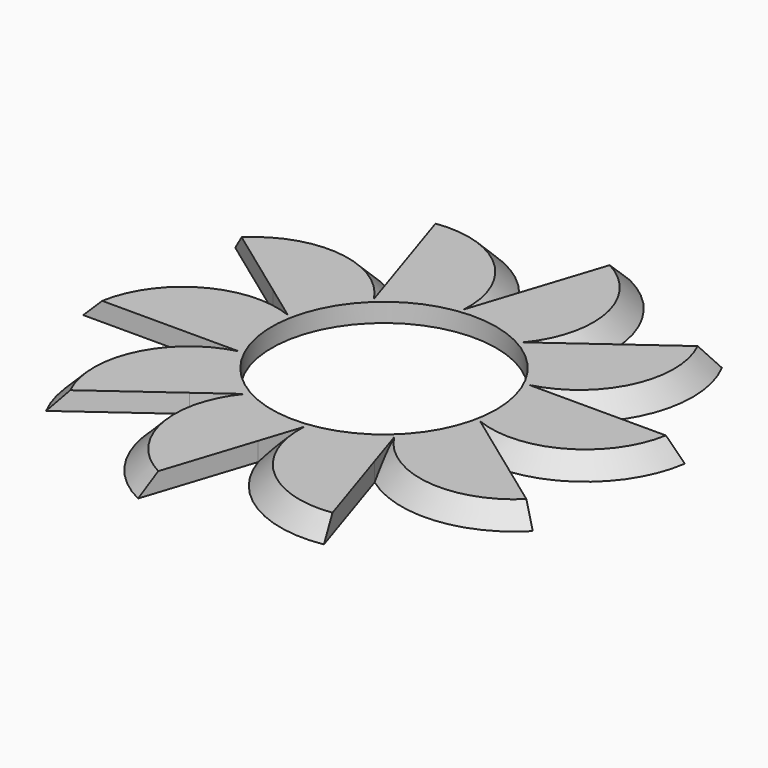
from build123d import *

# Parameters (mm, degrees)
F0_R         = 30
F1_DEPTH     = 5
F2_T4_ANGLE  = 130.4484876855
F2_T9_ANGLE  = 130.4484876855
F2_T14_ANGLE = 130.4484876855
F2_T19_ANGLE = 130.4484876855
F2_T24_ANGLE = 130.4484876855
F2_T29_ANGLE = 130.4484876855
F2_T34_ANGLE = 130.4484876855
F2_T39_ANGLE = 130.4484876855
F2_T44_ANGLE = 130.4484876855
F2_T49_ANGLE = 130.4484876855


# Not quite as in the source:
# - a fillet or chamfer that OpenCascade refuses, or shapes differently, is made with other operations: its cross-section is extruded or revolved along the edge and cut away or added


with BuildPart() as f1:
    # F0 (on Top) → F1 (new body)
    with BuildSketch(Plane.XY):
        with BuildLine():
            Line((-40, 12.9967878493), (-24.72135955, 34.0260323341))
            ThreePointArc((-24.72135955, 34.0260323341), (-45.1291822893, 39.7035462239), (-64.2705098312, 30.6303454181))
            Line((-64.2705098312, 30.6303454181), (-40, 12.9967878493))
        make_face()
        Polygon((40, -12.9967878493), (40, 12.9967878493), (24.72135955, 34.0260323341), (0, 42.0584889695), (-24.72135955, 34.0260323341), (-40, 12.9967878493), (-40, -12.9967878493), (-24.72135955, -34.0260323341), (0, -42.0584889695), (24.72135955, -34.0260323341), align=None)
        Circle(F0_R, mode=Mode.SUBTRACT)
        with BuildLine():
            Line((-24.72135955, 34.0260323341), (0, 42.0584889695))
            ThreePointArc((0, 42.0584889695), (-13.1731164802, 58.6471114297), (-33.9918693812, 62.5577278229))
            Line((-33.9918693812, 62.5577278229), (-24.72135955, 34.0260323341))
        make_face()
        with BuildLine():
            Line((0, 42.0584889695), (24.72135955, 34.0260323341))
            ThreePointArc((24.72135955, 34.0260323341), (23.8146320866, 55.1894734115), (9.2705098312, 70.5901844584))
            Line((9.2705098312, 70.5901844584), (0, 42.0584889695))
        make_face()
        with BuildLine():
            Line((24.72135955, 34.0260323341), (40, 12.9967878493))
            ThreePointArc((40, 12.9967878493), (51.7060006259, 30.6513323712), (48.9918693812, 51.6595899029))
            Line((48.9918693812, 51.6595899029), (24.72135955, 34.0260323341))
        make_face()
        with BuildLine():
            Line((70, 12.9967878493), (40, 12.9967878493))
            Line((40, 12.9967878493), (40, -12.9967878493))
            ThreePointArc((40, -12.9967878493), (59.8474343484, -5.5945758344), (70, 12.9967878493))
        make_face()
        with BuildLine():
            Line((64.2705098312, -30.6303454181), (40, -12.9967878493))
            Line((40, -12.9967878493), (24.72135955, -34.0260323341))
            ThreePointArc((24.72135955, -34.0260323341), (45.1291822893, -39.7035462239), (64.2705098312, -30.6303454181))
        make_face()
        with BuildLine():
            Line((33.9918693812, -62.5577278229), (24.72135955, -34.0260323341))
            Line((24.72135955, -34.0260323341), (0, -42.0584889695))
            ThreePointArc((0, -42.0584889695), (13.1731164802, -58.6471114297), (33.9918693812, -62.5577278229))
        make_face()
        with BuildLine():
            Line((-9.2705098312, -70.5901844584), (0, -42.0584889695))
            Line((0, -42.0584889695), (-24.72135955, -34.0260323341))
            ThreePointArc((-24.72135955, -34.0260323341), (-23.8146320866, -55.1894734115), (-9.2705098312, -70.5901844584))
        make_face()
        with BuildLine():
            Line((-48.9918693812, -51.6595899029), (-24.72135955, -34.0260323341))
            Line((-24.72135955, -34.0260323341), (-40, -12.9967878493))
            ThreePointArc((-40, -12.9967878493), (-51.7060006259, -30.6513323712), (-48.9918693812, -51.6595899029))
        make_face()
        with BuildLine():
            Line((-40, -12.9967878493), (-40, 12.9967878493))
            ThreePointArc((-40, 12.9967878493), (-59.8474343484, 5.5945758344), (-70, -12.9967878493))
            Line((-70, -12.9967878493), (-40, -12.9967878493))
        make_face()
    extrude(amount=F1_DEPTH)

    # F2: chamfer of 5 on 10 edges, made by hand


with BuildPart() as f2_tool2:
    # F2_s3 → F2_t4 (revolve)
    with BuildSketch(Plane(origin=(-19.7412033785, -21.6824721062, 0), x_dir=(0, 0, 1), z_dir=(0.6732302342, 0.7394329258, 0))):
        Polygon((0, 1.9388571331), (5, 6.9388571331), (5, 1.9388571331), align=None)
    revolve(axis=Axis((4.103379024, -43.3922083566, 5), (0, 0, 1)), revolution_arc=F2_T4_ANGLE)

    split(bisect_by=Plane(origin=(7.639320225, -10.5146222424, 0), x_dir=(0, 0, 1), z_dir=(0.5877852523, -0.8090169944, 0)), keep=Keep.TOP)


with BuildPart() as f1_1:
    add(f1.part)

    # F2_t1: cut F2_tool2
    add(f2_tool2.part, mode=Mode.SUBTRACT)


with BuildPart() as f2_tool7:
    # F2_s8 → F2_t9 (revolve)
    with BuildSketch(Plane(origin=(-28.7156063599, -5.9379002056, 0), x_dir=(0, 0, 1), z_dir=(0.9792824694, 0.2024990002, 0))):
        Polygon((0, 1.9388571331), (5, 6.9388571331), (5, 1.9388571331), align=None)
    revolve(axis=Axis((-22.1855967717, -37.5169396588, 5), (0, 0, 1)), revolution_arc=F2_T9_ANGLE)

    split(bisect_by=Plane.XZ.offset(12.9967878493), keep=Keep.TOP)


with BuildPart() as f1_2:
    add(f1_1.part)

    # F2_t6: cut F2_tool7
    add(f2_tool7.part, mode=Mode.SUBTRACT)


with BuildPart() as f2_tool12:
    # F2_s13 → F2_t14 (revolve)
    with BuildSketch(Plane(origin=(-26.7216237194, 12.0747477518, 0), x_dir=(0, 0, 1), z_dir=(0.911282086, -0.4117826609, 0))):
        Polygon((0, 1.9388571331), (5, 6.9388571331), (5, 1.9388571331), align=None)
    revolve(axis=Axis((-40.0004286612, -17.3114751652, 5), (0, 0, 1)), revolution_arc=F2_T14_ANGLE)

    split(bisect_by=Plane(origin=(-7.639320225, -10.5146222424, 0), x_dir=(0, 0, 1), z_dir=(-0.5877852523, -0.8090169944, 0)), keep=Keep.TOP)


with BuildPart() as f1_3:
    add(f1_2.part)

    # F2_t11: cut F2_tool12
    add(f2_tool12.part, mode=Mode.SUBTRACT)


with BuildPart() as f2_tool17:
    # F2_s18 → F2_t19 (revolve)
    with BuildSketch(Plane(origin=(-14.5208890526, 25.4752524735, 0), x_dir=(0, 0, 1), z_dir=(0.495202919, -0.8687773415, 0))):
        Polygon((0, 1.9388571331), (5, 6.9388571331), (5, 1.9388571331), align=None)
    revolve(axis=Axis((-42.5364563668, 9.5063844461, 5), (0, 0, 1)), revolution_arc=F2_T19_ANGLE)

    split(bisect_by=Plane(origin=(-12.360679775, -4.0162283177, 0), x_dir=(0, 0, 1), z_dir=(-0.9510565163, -0.3090169944, 0)), keep=Keep.TOP)


with BuildPart() as f1_4:
    add(f1_3.part)

    # F2_t16: cut F2_tool17
    add(f2_tool17.part, mode=Mode.SUBTRACT)


with BuildPart() as f2_tool22:
    # F2_s23 → F2_t24 (revolve)
    with BuildSketch(Plane(origin=(3.2263316853, 29.1450766224, 0), x_dir=(0, 0, 1), z_dir=(-0.1100269317, -0.9939286062, 0))):
        Polygon((0, 1.9388571331), (5, 6.9388571331), (5, 1.9388571331), align=None)
    revolve(axis=Axis((-28.8250035012, 32.6931283091, 5), (0, 0, 1)), revolution_arc=F2_T24_ANGLE)

    split(bisect_by=Plane(origin=(-12.360679775, 4.0162283177, 0), x_dir=(0, 0, 1), z_dir=(-0.9510565163, 0.3090169944, 0)), keep=Keep.TOP)


with BuildPart() as f1_5:
    add(f1_4.part)

    # F2_t21: cut F2_tool22
    add(f2_tool22.part, mode=Mode.SUBTRACT)


with BuildPart() as f2_tool27:
    # F2_s28 → F2_t29 (revolve)
    with BuildSketch(Plane(origin=(19.7412033785, 21.6824721062, 0), x_dir=(0, 0, 1), z_dir=(-0.6732302342, -0.7394329258, 0))):
        Polygon((0, 1.9388571331), (5, 6.9388571331), (5, 1.9388571331), align=None)
    revolve(axis=Axis((-4.103379024, 43.3922083566, 5), (0, 0, 1)), revolution_arc=F2_T29_ANGLE)

    split(bisect_by=Plane(origin=(-7.639320225, 10.5146222424, 0), x_dir=(0, 0, 1), z_dir=(-0.5877852523, 0.8090169944, 0)), keep=Keep.TOP)


with BuildPart() as f1_6:
    add(f1_5.part)

    # F2_t26: cut F2_tool27
    add(f2_tool27.part, mode=Mode.SUBTRACT)


with BuildPart() as f2_tool32:
    # F2_s33 → F2_t34 (revolve)
    with BuildSketch(Plane(origin=(28.7156063599, 5.9379002056, 0), x_dir=(0, 0, 1), z_dir=(-0.9792824694, -0.2024990002, 0))):
        Polygon((0, 1.9388571331), (5, 6.9388571331), (5, 1.9388571331), align=None)
    revolve(axis=Axis((22.1855967717, 37.5169396588, 5), (0, 0, 1)), revolution_arc=F2_T34_ANGLE)

    split(bisect_by=Plane.XZ.offset(-12.9967878493), keep=Keep.BOTTOM)


with BuildPart() as f1_7:
    add(f1_6.part)

    # F2_t31: cut F2_tool32
    add(f2_tool32.part, mode=Mode.SUBTRACT)


with BuildPart() as f2_tool37:
    # F2_s38 → F2_t39 (revolve)
    with BuildSketch(Plane(origin=(26.7216237194, -12.0747477518, 0), x_dir=(0, 0, 1), z_dir=(-0.911282086, 0.4117826609, 0))):
        Polygon((0, 1.9388571331), (5, 6.9388571331), (5, 1.9388571331), align=None)
    revolve(axis=Axis((40.0004286612, 17.3114751652, 5), (0, 0, 1)), revolution_arc=F2_T39_ANGLE)

    split(bisect_by=Plane(origin=(7.639320225, 10.5146222424, 0), x_dir=(0, 0, 1), z_dir=(0.5877852523, 0.8090169944, 0)), keep=Keep.TOP)


with BuildPart() as f1_8:
    add(f1_7.part)

    # F2_t36: cut F2_tool37
    add(f2_tool37.part, mode=Mode.SUBTRACT)


with BuildPart() as f2_tool42:
    # F2_s43 → F2_t44 (revolve)
    with BuildSketch(Plane(origin=(14.5208890526, -25.4752524735, 0), x_dir=(0, 0, 1), z_dir=(-0.495202919, 0.8687773415, 0))):
        Polygon((0, 1.9388571331), (5, 6.9388571331), (5, 1.9388571331), align=None)
    revolve(axis=Axis((42.5364563668, -9.5063844461, 5), (0, 0, 1)), revolution_arc=F2_T44_ANGLE)

    split(bisect_by=Plane(origin=(12.360679775, 4.0162283177, 0), x_dir=(0, 0, 1), z_dir=(0.9510565163, 0.3090169944, 0)), keep=Keep.TOP)


with BuildPart() as f1_9:
    add(f1_8.part)

    # F2_t41: cut F2_tool42
    add(f2_tool42.part, mode=Mode.SUBTRACT)


with BuildPart() as f2_tool47:
    # F2_s48 → F2_t49 (revolve)
    with BuildSketch(Plane(origin=(-3.2263316853, -29.1450766224, 0), x_dir=(0, 0, 1), z_dir=(0.1100269317, 0.9939286062, 0))):
        Polygon((0, 1.9388571331), (5, 6.9388571331), (5, 1.9388571331), align=None)
    revolve(axis=Axis((28.8250035012, -32.6931283091, 5), (0, 0, 1)), revolution_arc=F2_T49_ANGLE)

    split(bisect_by=Plane(origin=(12.360679775, -4.0162283177, 0), x_dir=(0, 0, 1), z_dir=(0.9510565163, -0.3090169944, 0)), keep=Keep.TOP)


with BuildPart() as f1_10:
    add(f1_9.part)

    # F2_t46: cut F2_tool47
    add(f2_tool47.part, mode=Mode.SUBTRACT)


solid = f1_10.part
